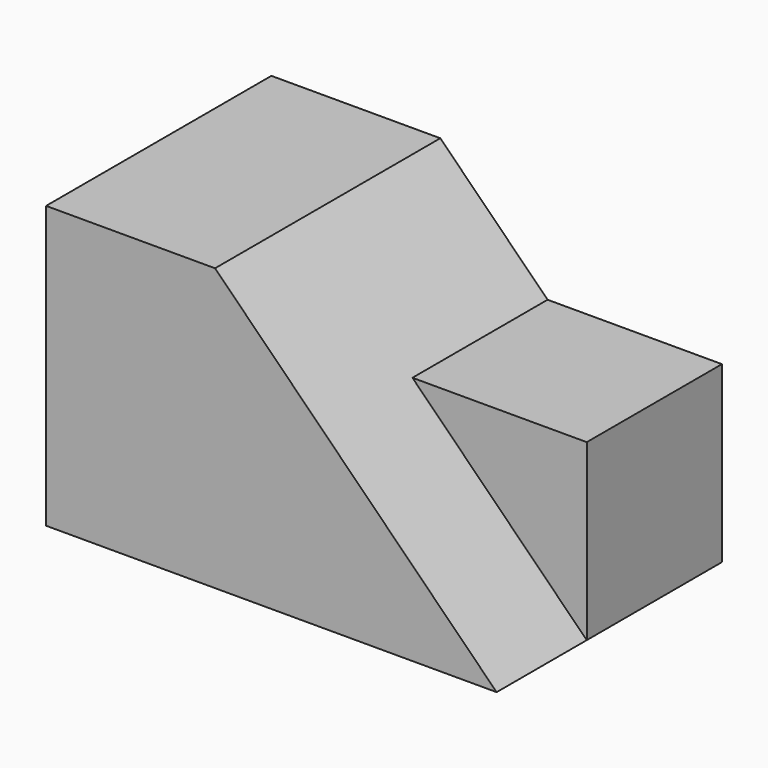
from build123d import *

# Parameters (mm, degrees)
F0_W     = 50.8
F0_H     = 31.75
F1_DEPTH = 31.75
F3_DEPTH = 31.75
F5_DEPTH = 19.05


# Not quite as in the source:
# - a length typed as a fraction of an inch, garbled in the dataset ("3 / 203.2 mm" for 3/8 in), is restored


with BuildPart() as f1:
    # F0 (on Front) → F1 (new body)
    with BuildSketch(Plane.XZ):
        with Locations((25.4, 15.875)):
            Rectangle(F0_W, F0_H)
    extrude(amount=F1_DEPTH)

    # F2 (on face) → F3 (cut)
    with BuildSketch(Plane.XZ.offset(31.75)):
        Polygon((19.05, 31.75), (50.8, 0), (50.8, 31.75), align=None)
    extrude(amount=-F3_DEPTH, mode=Mode.SUBTRACT)

    # F4 (on face) → F5 (join)
    with BuildSketch(Plane(origin=(0, 0, 0), x_dir=(-1, 0, 0), z_dir=(0, 1, 0))):
        Polygon((-50.8, 19.6542944759), (-50.8, 0), (-31.1457055241, 19.6542944759), align=None)
    extrude(amount=-F5_DEPTH)


solid = f1.part
